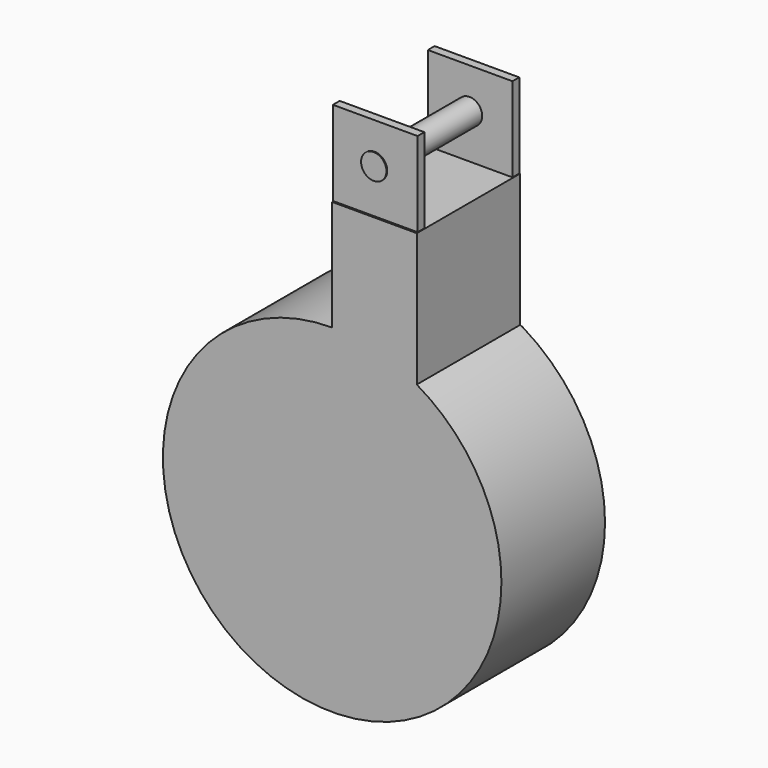
from build123d import *

# Parameters (mm, degrees)
F0_R     = 50.8
F1_DEPTH = 38.862
F2_W     = 38.7112945318
F2_H     = 79.9200646579
F4_DEPTH = 25.4
F5_W     = 2.54
F5_H     = 25.4
F6_DEPTH = 25.4
F7_R     = 3.81
F8_DEPTH = 36.83


# Not quite as in the source:
# - the program builds the solid bodies; features that only make, move or delete a surface that nothing else refers to are left out


with BuildPart() as f1:
    # F0 (on Front) → F1 (new body)
    with BuildSketch(Plane.XZ):
        Circle(F0_R)
    extrude(amount=-F1_DEPTH)

    # F2 (on Right) → F4 (join)
    with BuildSketch(Plane.YZ):
        with Locations((19.3556472659, 44.0184753388)):
            Rectangle(F2_W, F2_H)
    extrude(amount=F4_DEPTH)


with BuildPart() as f6:
    # F5 (on Right) → F6 (new body)
    with BuildSketch(Plane.YZ):
        with Locations((1.5609483235, 96.833985544)):
            Rectangle(F5_W, F5_H)
    extrude(amount=F6_DEPTH)


with BuildPart() as f6b:
    # F5 (on Right) → F6, piece 2 (new body)
    with BuildSketch(Plane.YZ):
        with Locations((37.1715911818, 96.833985544)):
            Rectangle(F5_W, F5_H)
    extrude(amount=F6_DEPTH)


with BuildPart() as f8:
    # F7 (on Front) → F8 (new body)
    with BuildSketch(Plane.XZ):
        with Locations((12.4874990433, 97.4025800824)):
            Circle(F7_R)
    extrude(amount=-F8_DEPTH)


solid = Compound([f1.part, f6.part, f6b.part, f8.part])
